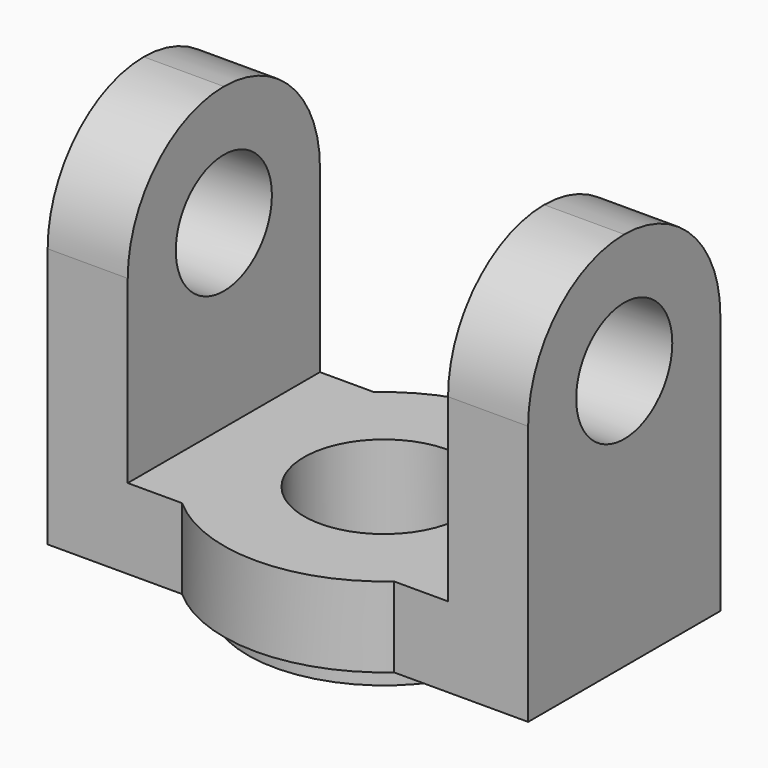
from build123d import *

# Parameters (mm, degrees)
F1_DEPTH  = 47.5
F2_W      = 40
F2_H      = 37.5
F3_DEPTH  = 205
F4_W      = 26.4575131106
F4_H      = 37.5
F5_DEPTH  = 25
F6_R      = 17
F7_DEPTH  = 3
F8_R      = 10
F9_DEPTH  = 25
F11_DEPTH = 125
F12_R     = 14.99999


# Not quite as in the source:
# - a fillet or chamfer is up to 0.001 mm smaller than in the source, because OpenCascade refuses the exact size


with BuildPart() as f1:
    # F0 (on Top) → F1 (new body)
    with BuildSketch(Plane.XY):
        Polygon((0, 15), (0, 0), (16.7712434447, 0), (43.2287565553, 0), (60, 0), (60, 15), (60, 30), (43.2287565553, 30), (16.7712434447, 30), (0, 30), align=None)
        with BuildLine():
            Line((49.2664991614, 20.3667504193), (60, 15))
            Line((60, 15), (50, 15))
            ThreePointArc((50, 15), (49.8157763314, 17.7083220609), (49.2664991614, 20.3667504193))
        make_face(mode=Mode.SUBTRACT)
        with BuildLine():
            Line((43.2287565553, 0), (16.7712434447, 0))
            ThreePointArc((16.7712434447, 0), (30, -5), (43.2287565553, 0))
        make_face()
        with BuildLine():
            ThreePointArc((43.2287565553, 30), (30, 35), (16.7712434447, 30))
            Line((16.7712434447, 30), (43.2287565553, 30))
        make_face()
        with BuildLine():
            Line((50, 15), (60, 15))
            Line((60, 15), (49.2664991614, 20.3667504193))
            ThreePointArc((49.2664991614, 20.3667504193), (49.8157763314, 17.7083220609), (50, 15))
        make_face()
    extrude(amount=F1_DEPTH)

    # F2 (on face) → F3 (cut)
    with BuildSketch(Plane.XZ):
        with Locations((30, 28.75)):
            Rectangle(F2_W, F2_H)
    extrude(amount=-F3_DEPTH, mode=Mode.SUBTRACT)

    # F4 (on face) → F5 (cut)
    with BuildSketch(Plane(origin=(0, 0, 0), x_dir=(-1, 0, 0), z_dir=(0, 1, 0))):
        with Locations((-30, 28.75)):
            Rectangle(F4_W, F4_H)
    extrude(amount=-F5_DEPTH, mode=Mode.SUBTRACT)

    # F6 (on face) → F7 (join)
    with BuildSketch(Plane(origin=(0, 0, 0), x_dir=(1, 0, 0), z_dir=(0, 0, -1))):
        with Locations((30, -15)):
            Circle(F6_R)
    extrude(amount=F7_DEPTH)

    # F8 (on face) → F9 (cut)
    with BuildSketch(Plane(origin=(0, 0, -3), x_dir=(1, 0, 0), z_dir=(0, 0, -1))):
        with Locations((30, -15)):
            Circle(F8_R)
    extrude(amount=-F9_DEPTH, mode=Mode.SUBTRACT)

    # F10 (on face) → F11 (cut)
    with BuildSketch(Plane.YZ.offset(60)):
        with BuildLine():
            ThreePointArc((15, 25), (20.3033008589, 27.1966991411), (22.5, 32.5))
            ThreePointArc((22.5, 32.5), (9.6966991411, 37.8033008589), (15, 25))
        make_face()
    extrude(amount=-F11_DEPTH, mode=Mode.SUBTRACT)

    # F12 (radius 15 in the source; OpenCascade refuses exactly that, so slightly less here)
    f12_edges = [f1.edges().sort_by_distance(p)[0] for p in [
        (55, 0, 47.5),
        (55, 30, 47.5),
        (5, 0, 47.5),
        (5, 30, 47.5),
    ]]
    fillet(f12_edges, radius=F12_R)


solid = f1.part
